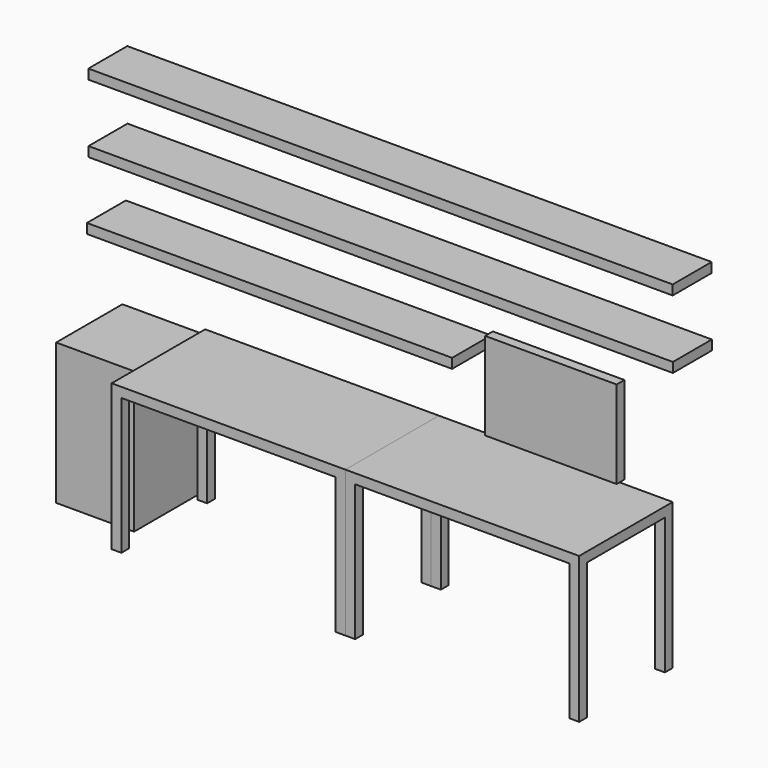
from build123d import *

# Parameters (mm, degrees)
F0_W     = 3048
F0_H     = 50.8
F1_DEPTH = 254
F0_W_2   = 1905
F0_W_3   = 1219.2
F2_DEPTH = 609.6
F3_START = 101.6
F0_W_4   = 685.8
F0_H_2   = 457.2
F3_DEPTH = 50.8
F4_DEPTH = 609.6
F5_W     = 50.8
F5_H     = 50.8
F6_DEPTH = 711.2
F7_DEPTH = 711.2
F0_W_5   = 406.4
F0_H_3   = 736.6
F8_DEPTH = 431.8


with BuildPart() as f1:
    # F0 (on Front) → F1 (new body)
    with BuildSketch(Plane.XZ):
        with Locations((0.2425422668, 1905)):
            Rectangle(F0_W, F0_H)
    extrude(amount=F1_DEPTH)


with BuildPart() as f1b:
    # F0 (on Front) → F1, piece 2 (new body)
    with BuildSketch(Plane.XZ):
        with Locations((1.1422147751, 1549.4)):
            Rectangle(F0_W, F0_H)
    extrude(amount=F1_DEPTH)


with BuildPart() as f1c:
    # F0 (on Front) → F1, piece 3 (new body)
    with BuildSketch(Plane.XZ):
        with Locations((-578.7231035233, 1193.8)):
            Rectangle(F0_W_2, F0_H)
    extrude(amount=F1_DEPTH)


with BuildPart() as f2:
    # F0 (on Front) → F2 (new body)
    with BuildSketch(Plane.XZ):
        with Locations((-508, 736.6)):
            Rectangle(F0_W_3, F0_H)
    extrude(amount=F2_DEPTH)

    # F5 (on face) → F6 (join)
    with BuildSketch(Plane(origin=(0, 0, 711.2), x_dir=(1, 0, 0), z_dir=(0, 0, -1))):
        with Locations((76.2, 584.2)):
            Rectangle(F5_W, F5_H)
        with Locations((-1092.2, 584.2)):
            Rectangle(F5_W, F5_H)
        with Locations((-1092.2, 25.4)):
            Rectangle(F5_W, F5_H)
        with Locations((76.2, 25.4)):
            Rectangle(F5_W, F5_H)
    extrude(amount=F6_DEPTH)


with BuildPart() as f3:
    # F0 (on Front) → F3 (new body)
    with BuildSketch(Plane.XZ.offset(F3_START)):
        with Locations((807.2379013062, 1079.5)):
            Rectangle(F0_W_4, F0_H_2)
    extrude(amount=F3_DEPTH)


with BuildPart() as f4:
    # F0 (on Front) → F4 (new body)
    with BuildSketch(Plane.XZ):
        with Locations((711.2, 736.6)):
            Rectangle(F0_W_3, F0_H)
    extrude(amount=F4_DEPTH)

    # F5 (on face) → F7 (join)
    with BuildSketch(Plane(origin=(0, 0, 711.2), x_dir=(1, 0, 0), z_dir=(0, 0, -1))):
        with Locations((127, 584.2)):
            Rectangle(F5_W, F5_H)
        with Locations((127, 25.4)):
            Rectangle(F5_W, F5_H)
        with Locations((1295.4, 584.2)):
            Rectangle(F5_W, F5_H)
        with Locations((1295.4, 25.4)):
            Rectangle(F5_W, F5_H)
    extrude(amount=F7_DEPTH)


with BuildPart() as f8:
    # F0 (on Front) → F8 (new body)
    with BuildSketch(Plane.XZ):
        with Locations((-1346.2, 368.3)):
            Rectangle(F0_W_5, F0_H_3)
    extrude(amount=F8_DEPTH)


solid = Compound([f1.part, f1b.part, f1c.part, f2.part, f3.part, f4.part, f8.part])
